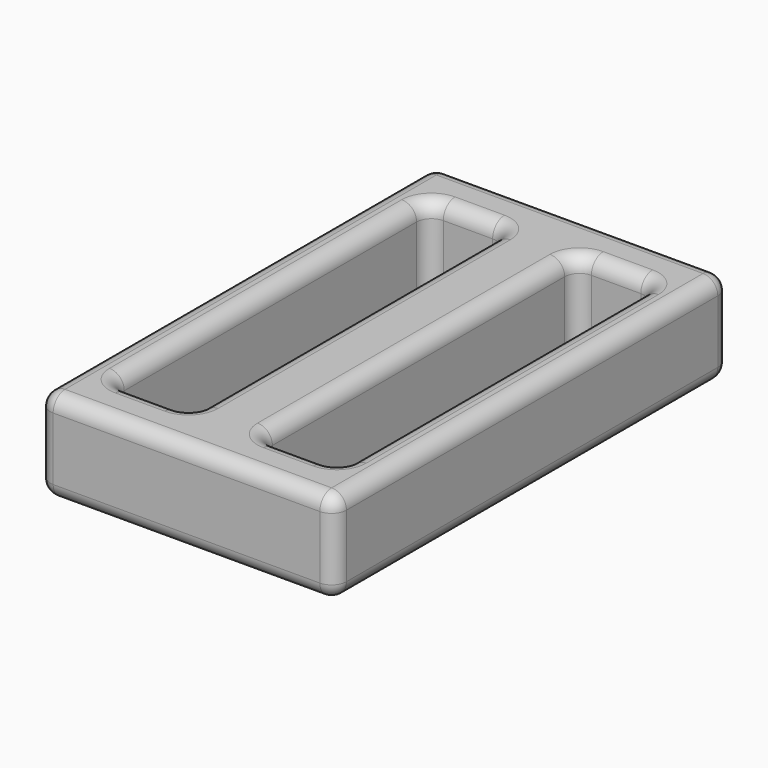
from build123d import *

# Parameters (mm, degrees)
F0_W     = 15.24
F0_H     = 25.4
F1_DEPTH = 4.7625
F2_W     = 4.064
F2_H     = 20.32
F3_DEPTH = 25.4
F4_R     = 0.762


# Not quite as in the source:
# - a pattern or mirror of a feature is missing from the dataset's text; its kind, count and spacing are read off the source's solid
# - the program builds the solid bodies; features that only make, move or delete a surface that nothing else refers to are left out


with BuildPart() as f1:
    # F0 (on Top) → F1 (new body)
    with BuildSketch(Plane.XY):
        Rectangle(F0_W, F0_H)
    extrude(amount=F1_DEPTH)

    # F2 (on face) → F3 (cut)
    with BuildSketch(Plane.XY.offset(4.7625)):
        with Locations((3.81, 0)):
            Rectangle(F2_W, F2_H)
    f3 = extrude(amount=-F3_DEPTH, mode=Mode.SUBTRACT)

    # F3_copies: F3 across plane
    add(f3.mirror(Plane(origin=(0, 0, 0), x_dir=(0, 0, -1), z_dir=(-1, 0, 0))), mode=Mode.SUBTRACT)

    # F4
    f4_edges = [f1.edges().sort_by_distance(p)[0] for p in [
        (0, -12.7, 4.7625),
        (-7.62, 0, 4.7625),
        (7.62, 0, 4.7625),
        (0, 12.7, 4.7625),
        (-1.778, 0, 4.7625),
        (-3.81, 10.16, 4.7625),
        (-5.842, 0, 4.7625),
        (-3.81, -10.16, 4.7625),
        (3.81, -10.16, 4.7625),
        (1.778, 0, 4.7625),
        (5.842, 0, 4.7625),
        (3.81, 10.16, 4.7625),
        (0, -12.7, 0),
        (-7.62, 0, 0),
        (7.62, 0, 0),
        (0, 12.7, 0),
        (-1.778, 0, 0),
        (-3.81, 10.16, 0),
        (-5.842, 0, 0),
        (-3.81, -10.16, 0),
        (3.81, -10.16, 0),
        (1.778, 0, 0),
        (5.842, 0, 0),
        (3.81, 10.16, 0),
        (-7.62, -12.7, 2.38125),
        (7.62, -12.7, 2.38125),
        (7.62, 12.7, 2.38125),
        (-7.62, 12.7, 2.38125),
        (5.842, 10.16, 2.38125),
        (5.842, -10.16, 2.38125),
        (1.778, -10.16, 2.38125),
        (1.778, 10.16, 2.38125),
        (-1.778, -10.16, 2.38125),
        (-1.778, 10.16, 2.38125),
        (-5.842, 10.16, 2.38125),
        (-5.842, -10.16, 2.38125),
    ]]
    fillet(f4_edges, radius=F4_R)


solid = f1.part
